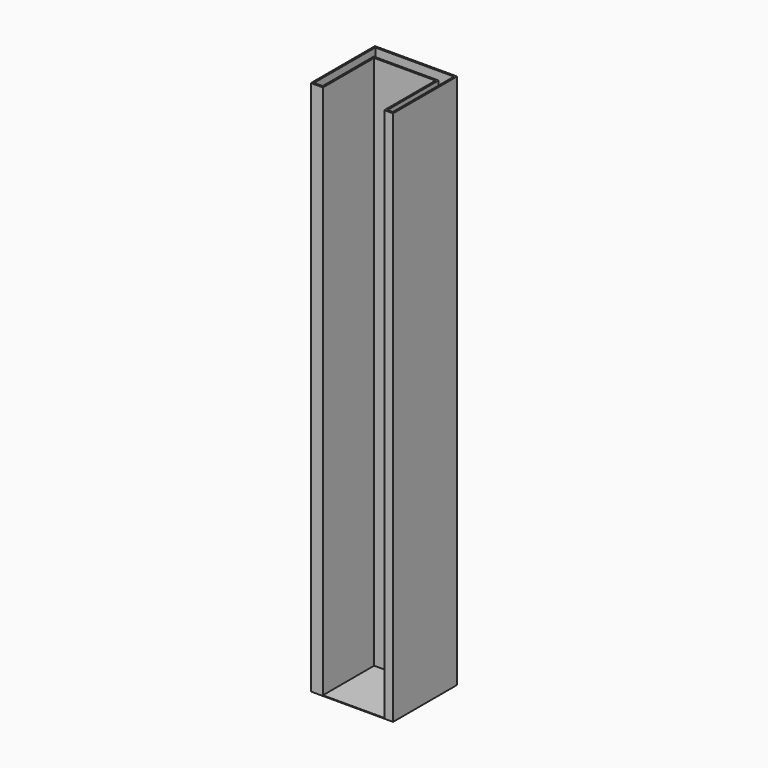
from build123d import *

# Parameters (mm, degrees)
F0_W        = 120.9424138069
F0_H        = 117.7590936422
F1_DEPTH    = 1
F4_DEPTH    = 25.4
F5_DEPTH    = 762
F6_T        = 2.54
F6_T3_DEPTH = 792.48
F6_T5_DEPTH = 99.200644033
F6_T7_DEPTH = 95.3667019176


# Not quite as in the source:
# - a shell that OpenCascade refuses in one call is made with other operations: the cavity is built on its own and cut out


with BuildPart() as f1:
    # F0 (on Top) → F1 (new body)
    with BuildSketch(Plane.XY):
        Rectangle(F0_W, F0_H)
    extrude(amount=F1_DEPTH)

    # F3 (on face) → F4 (join)
    with BuildSketch(Plane.XY.offset(1)):
        Polygon((-60.4712069035, 58.8795468211), (-60.4712069035, -58.8795468211), (-42.7266806364, -58.8795468211), (-42.7266806364, 35.2410972118), (47.5600212812, 35.2410972118), (47.5600212812, -58.8795468211), (60.4712069035, -58.8795468211), (60.4712069035, 58.8795468211), align=None)
    extrude(amount=F4_DEPTH)

    # F5 (add): a face of the model
    f5_faces = [f1.faces().sort_by_distance(p)[0] for p in [
        (-58.7831822711, 0, 26.4),
    ]]
    extrude(f5_faces, amount=F5_DEPTH)

    # F6: shell of thickness 2.54, made by hand


with BuildPart() as f6_core1:
    # F6_t2: copy of F1
    add(f1.part)

    # the walls: a layer under each face that stays
    f6_faces = [f6_core1.faces().sort_by_distance(p)[0] for p in [
        (0, 58.8795468211, 394.2),
        (0, 0, 0),
        (-51.8324630601, -58.8795468211, 732.0857142857),
        (47.5600212812, -11.8192248046, 394.7),
        (2.4166703224, 35.2410972118, 394.7),
        (2.4166703224, -11.8192248046, 1),
        (-42.7266806364, -11.8192248046, 394.7),
        (-60.4712069035, 0, 394.2),
        (60.4712069035, 0, 394.2),
    ]]
    thicken(f6_faces, amount=-F6_T, mode=Mode.SUBTRACT)

    # F6_s4 → F6_t3 (cut)
    with BuildSketch(Plane.XY.offset(-1.54)):
        Polygon((47.5346212812, 35.2156972118), (50.1000212812, 35.2410972118), (50.1000212812, 37.7810972118), (47.5600212812, 37.7810972118), align=None)
        Polygon((-42.7012806364, 35.2156972118), (-42.7266806364, 37.7810972118), (-45.2666806364, 37.7810972118), (-45.2666806364, 35.2410972118), align=None)
    extrude(amount=F6_T3_DEPTH, mode=Mode.SUBTRACT)

    # F6_s6 → F6_t5 (cut)
    with BuildSketch(Plane.XZ.offset(-37.7810972118)):
        Polygon((47.5346212812, 1.0254), (50.1000212812, 1), (50.1000212812, -1.54), (47.5600212812, -1.54), align=None)
        Polygon((-42.7012806364, 1.0254), (-42.7266806364, -1.54), (-45.2666806364, -1.54), (-45.2666806364, 1), align=None)
    extrude(amount=F6_T5_DEPTH, mode=Mode.SUBTRACT)

    # F6_s8 → F6_t7 (cut)
    with BuildSketch(Plane.YZ.offset(-45.2666806364)):
        Polygon((35.2156972118, 1.0254), (37.7810972118, 1), (37.7810972118, -1.54), (35.2410972118, -1.54), align=None)
    extrude(amount=F6_T7_DEPTH, mode=Mode.SUBTRACT)


with BuildPart() as f1_1:
    add(f1.part)

    # what is left inside the walls is the cavity
    f6_cavity = [f6_core1.part.solids().sort_by_distance(p)[0] for p in [
        (0, 56.314147, 526.446667),
    ]]
    add(f6_cavity, mode=Mode.SUBTRACT)


solid = f1_1.part
